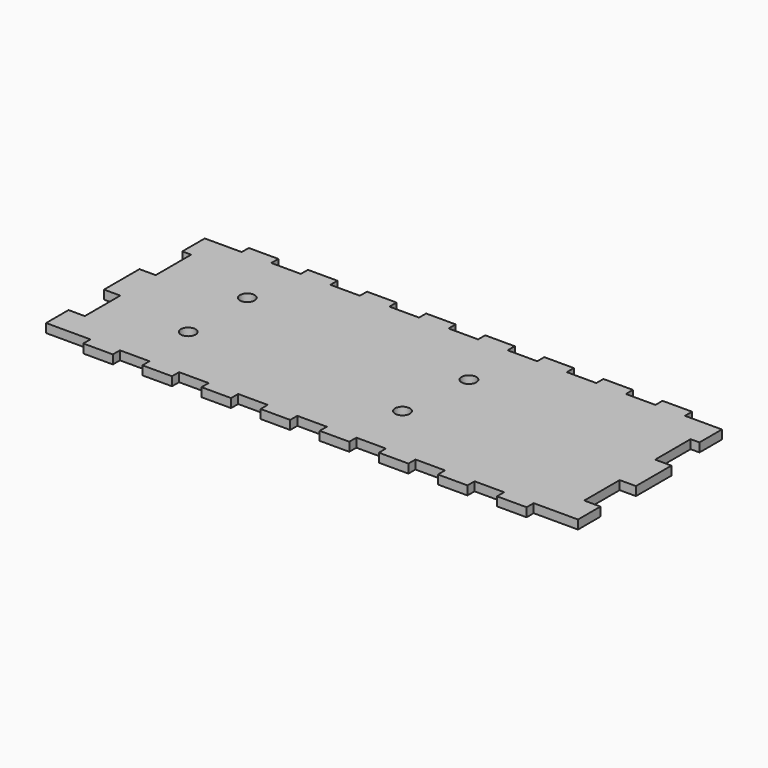
from build123d import *

# Parameters (mm, degrees)
F0_R     = 2.5
F1_DEPTH = 3


# Not quite as in the source:
# - ends of sketch curves that miss each other by under 0.0002 mm in the source are joined


with BuildPart() as f1:
    # F0 (on Top) → F1 (new body)
    with BuildSketch(Plane.XY):
        Polygon((-34.5, 32), (-47, 32), (-47, 22.4999984801), (-44, 22.4999984801), (-44, 7.4999984801), (-49.5, 7.4999984801), (-49.5, -7.5000015199), (-44, -7.5000015199), (-44, -22.5000015199), (-49.5, -22.5000015199), (-49.5, -32.0000015199), (-34.5, -32), (-34.5, -35), (-24.5, -35), (-24.5, -32), (-14.5, -32), (-14.5, -35), (-4.5, -35), (-4.5, -32), (5.5, -32), (5.5, -35), (15.5, -35), (15.5, -32), (25.5, -32), (25.5, -35), (35.5, -35), (35.5, -32), (40.5, -32), (45.5, -32), (45.5, -35), (55.5, -35), (55.5, -32), (65.5, -32), (65.5, -35), (75.5, -35), (75.5, -32), (85.5, -32), (85.5, -35), (95.5, -35), (95.5, -32), (105.5, -32), (105.5, -35), (115.5, -35), (115.5, -32), (130.5, -32), (130.5, -22.5000015199), (125, -22.5000015199), (125, -7.5000015199), (130.5, -7.5000015199), (130.5, 7.4999984801), (125, 7.4999984801), (125, 22.4999984801), (128, 22.4999984801), (128, 31.9999984801), (115.5, 32), (115.5, 35), (105.5, 35), (105.5, 32), (95.5, 32), (95.5, 35), (85.5, 35), (85.5, 32), (75.5, 32), (75.5, 35), (65.5, 35), (65.5, 32), (55.5, 32), (55.5, 35), (45.5, 35), (45.5, 32), (40.5, 32), (35.5, 32), (35.5, 35), (25.5, 35), (25.5, 32), (15.5, 32), (15.5, 35), (5.5, 35), (5.5, 32), (-4.5, 32), (-4.5, 35), (-14.5, 35), (-14.5, 32), (-24.5, 32), (-24.5, 35), (-34.5, 35), align=None)
        with Locations((-17, -12.5)):
            Circle(F0_R, mode=Mode.SUBTRACT)
        with Locations((55.5, -12.5)):
            Circle(F0_R, mode=Mode.SUBTRACT)
        with Locations((-17, 12.5)):
            Circle(F0_R, mode=Mode.SUBTRACT)
        with Locations((58, 12.5)):
            Circle(F0_R, mode=Mode.SUBTRACT)
    extrude(amount=F1_DEPTH)


solid = f1.part
